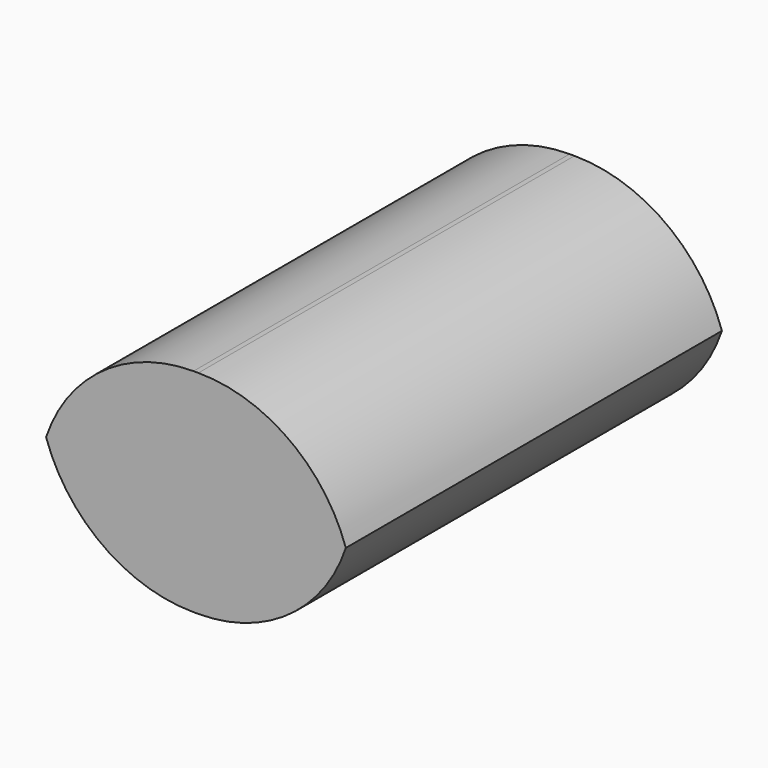
from build123d import *

# Parameters (mm, degrees)
F0_W        = 27.7576074004
F0_H        = 41.3104146719
F1_DEPTH    = 18.6459105462
F2_T1_DEPTH = 109.6348425509


# Not quite as in the source:
# - a fillet or chamfer that OpenCascade refuses, or shapes differently, is made with other operations: its cross-section is extruded or revolved along the edge and cut away or added


with BuildPart() as f1:
    # F0 (on Top) → F1 (new body)
    with BuildSketch(Plane.XY):
        with Locations((27.7516692877, -49.2671057582)):
            Rectangle(F0_W, F0_H)
    extrude(amount=F1_DEPTH)

    # F2: fillet of radius 13.6648855758 on 4 edges, made by hand

    # F2_s2 → F2_t1 (cut)
    with BuildSketch(Plane.XZ.offset(-5.5503155173)):
        with BuildLine():
            ThreePointArc((41.6304729879, 4.9810249704), (37.6281206669, 14.6435582252), (27.9655874121, 18.6459105462))
            Line((27.9655874121, 18.6459105462), (41.6304729879, 18.6459105462))
            Line((41.6304729879, 18.6459105462), (41.6304729879, 4.9810249704))
        make_face()
        with BuildLine():
            ThreePointArc((13.8728655875, 4.9810249704), (17.8752179085, 14.6435582252), (27.5377511633, 18.6459105462))
            Line((27.5377511633, 18.6459105462), (13.8728655875, 18.6459105462))
            Line((13.8728655875, 18.6459105462), (13.8728655875, 4.9810249704))
        make_face()
        with BuildLine():
            ThreePointArc((41.6304729879, 13.6648855758), (37.6281206669, 4.002352321), (27.9655874121, 0))
            Line((27.9655874121, 0), (41.6304729879, 0))
            Line((41.6304729879, 0), (41.6304729879, 13.6648855758))
        make_face()
        with BuildLine():
            ThreePointArc((13.8728655875, 13.6648855758), (17.8752179085, 4.002352321), (27.5377511633, 0))
            Line((27.5377511633, 0), (13.8728655875, 0))
            Line((13.8728655875, 0), (13.8728655875, 13.6648855758))
        make_face()
    extrude(amount=F2_T1_DEPTH, mode=Mode.SUBTRACT)


solid = f1.part
